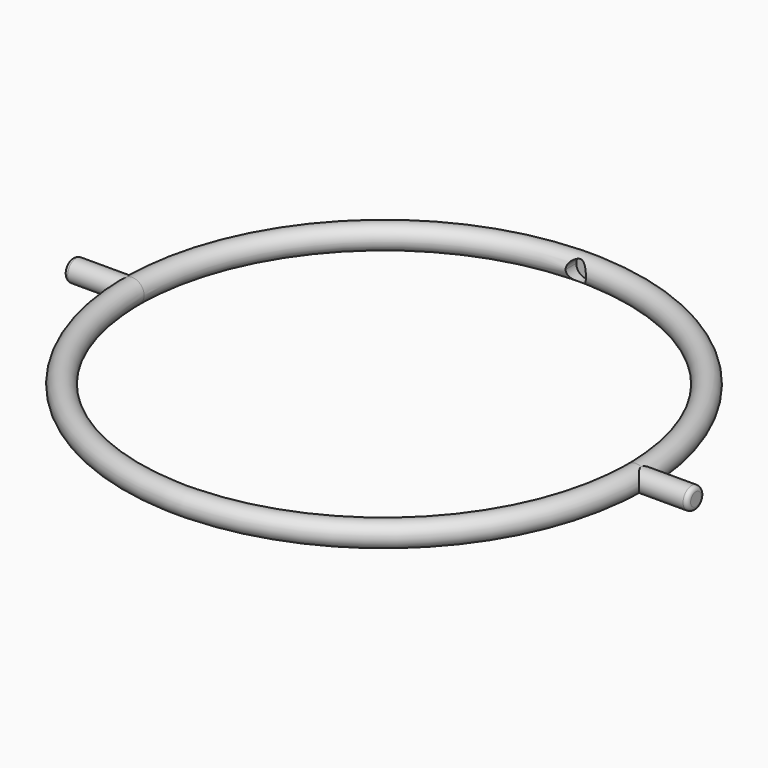
from build123d import *
from build123d import SkipClean  # not in build123d's __all__

# Parameters (mm, degrees)
F1_R     = 2.54
F4_R     = 2.159
F5_DEPTH = 4.064
F7_R     = 2.286
F8_DEPTH = 4.064
F10_R    = 2.286
F12_R    = 0.889


with BuildPart() as f2:
    # F2: sweep along a path in F0
    with BuildLine(Plane.XY) as f2_path:
        CenterArc((0, 0), 53.34, 0, 360)
    # F1 (on Right) → F2 (sweep)
    with BuildSketch(Plane.YZ):
        with Locations((-53.34, 0)):
            Circle(F1_R)
    sweep(path=f2_path.line)

    # F4 (on offset) → F5 (cut)
    with BuildSketch(Plane.XZ.offset(-49.53)):
        Circle(F4_R)
    extrude(amount=-F5_DEPTH, mode=Mode.SUBTRACT)

    # F7 (on offset) → F8 (cut)
    with BuildSketch(Plane.XZ.offset(49.53)):
        Circle(F7_R)
    extrude(amount=F8_DEPTH, mode=Mode.SUBTRACT)

    # F10 (on offset) → F11 (join, up to the next surface of F2)
    with BuildSketch(Plane.YZ.offset(66.04)):
        Circle(F10_R)
    extrude(until=Until.NEXT, dir=(-1, 0, 0))

    # F12
    f12_edges = [f2.edges().sort_by_distance(p)[0] for p in [
        (66.04, -2.286, 0),
    ]]
    fillet(f12_edges, radius=F12_R)

    # F13: F2 across plane


with BuildPart() as f2_1:
    add(f2.part, clean=False)
    with SkipClean():  # cleaning this boolean's faces spoils the solid; the shape is the same uncleaned
        add(f2.part.mirror(Plane.YZ), clean=False)


solid = f2_1.part
